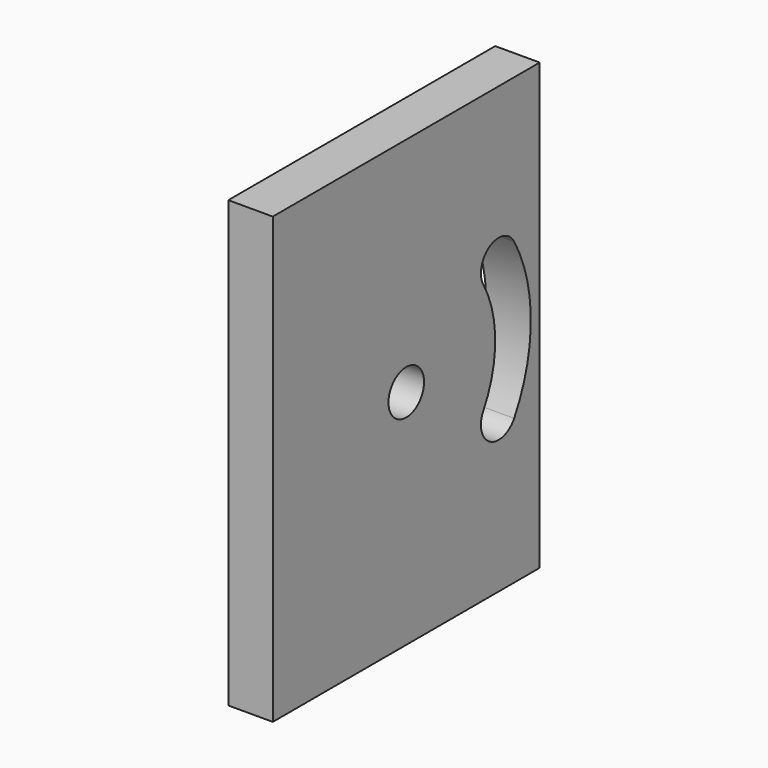
from build123d import *

# Parameters (mm, degrees)
F0_W     = 10
F0_H     = 75
F1_DEPTH = 100
F3_D     = 5
F3_DEPTH = 15
F3_TIP   = 1.5021515476
F4_R     = 5
F5_DEPTH = 10
F7_DEPTH = 10


with BuildPart() as f1:
    # F0 (on Top) → F1 (new body)
    with BuildSketch(Plane.XY):
        Rectangle(F0_W, F0_H)
    extrude(amount=F1_DEPTH)

    # F3
    with Locations(Plane(origin=(0, 0, 0), x_dir=(1, 0, 0), z_dir=(0, 0, -1))):
        with Locations((0, 25), (0, -25)):
            Hole(F3_D / 2, depth=F3_DEPTH)
            with Locations((0, 0, -(F3_DEPTH + F3_TIP / 2))):  # 118° drill point
                Cone(0, F3_D / 2, F3_TIP, mode=Mode.SUBTRACT)

    # F4 (on face) → F5 (cut, through all)
    with BuildSketch(Plane(origin=(-5, 0, 0), x_dir=(0, -1, 0), z_dir=(-1, 0, 0))):
        with Locations((0, 50)):
            Circle(F4_R)
    extrude(amount=-F5_DEPTH, mode=Mode.SUBTRACT)

    # F6 (on face) → F7 (cut, through all)
    with BuildSketch(Plane(origin=(-5, 0, 0), x_dir=(0, -1, 0), z_dir=(-1, 0, 0))):
        with BuildLine():
            ThreePointArc((-21.6506350946, 37.5), (-25, 50), (-21.6506350946, 62.5))
            ThreePointArc((-21.6506350946, 62.5), (-23.4807621135, 69.3301270189), (-30.3108891325, 67.5))
            ThreePointArc((-30.3108891325, 67.5), (-35, 50), (-30.3108891325, 32.5))
            ThreePointArc((-30.3108891325, 32.5), (-23.4807621135, 30.6698729811), (-21.6506350946, 37.5))
        make_face()
    extrude(amount=-F7_DEPTH, mode=Mode.SUBTRACT)


solid = f1.part
